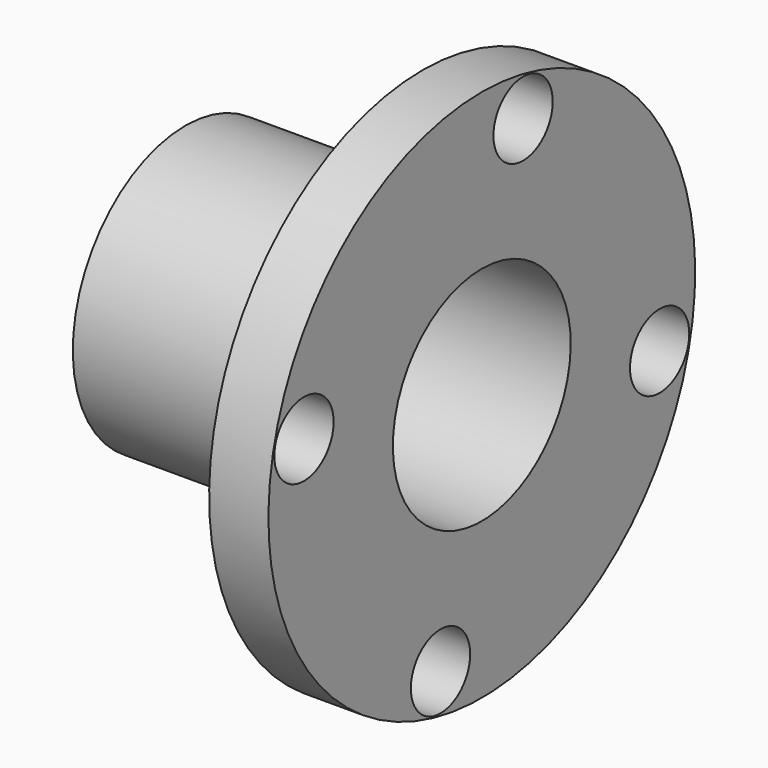
from build123d import *

# Parameters (mm, degrees)
F2_R            = 12.5
F3_DEPTH        = 20.001
F3_COPIES_COUNT = 4


# Not quite as in the source:
# - a pattern or mirror of a feature is missing from the dataset's text; its kind, count and spacing are read off the source's solid


with BuildPart() as f1:
    # F0 (on Front) → F1 (revolve)
    with BuildSketch(Plane.XZ):
        Polygon((-33.186925382, 90), (-53.186925382, 90), (-53.186925382, 47.5), (-133.186925382, 47.5), (-133.186925382, 37.5), (-33.186925382, 37.5), align=None)
    revolve(axis=Axis((-80.5058263218, 0, 0), (-1, 0, 0)))

    # F2 (on face) → F3 (cut, through all)
    with BuildSketch(Plane(origin=(-53.186925382, 0, 0), x_dir=(0, -1, 0), z_dir=(-1, 0, 0))):
        with Locations((75, 17.4127053469)):
            Circle(F2_R)
    f3 = extrude(amount=-F3_DEPTH, mode=Mode.SUBTRACT)

    # F3_copies: F3 ×4 about axis
    f3_copies_axis = Axis((0, 0, 0), (1, 0, 0))
    for i in range(1, F3_COPIES_COUNT):
        add(f3.rotate(f3_copies_axis, i * 360 / F3_COPIES_COUNT), mode=Mode.SUBTRACT)


solid = f1.part
